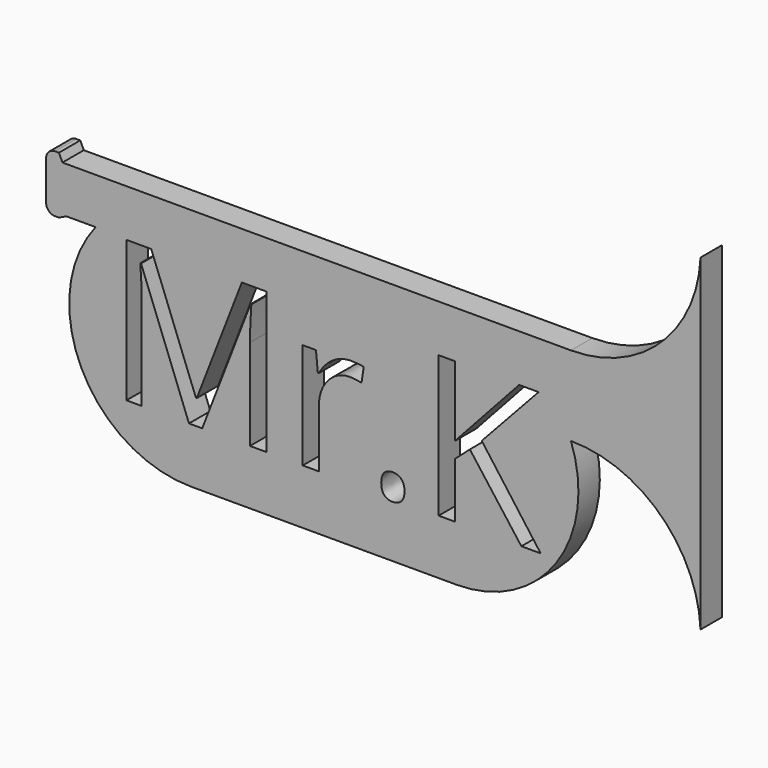
from build123d import *

# Parameters (mm, degrees)
F1_DEPTH     = 3
F2_TEXT_SIZE = 22.2222222222
F3_DEPTH     = 25


# Not quite as in the source:
# - Text() gives the source's letters only with a copy of the font that has no kerning and outlines rounded to 1/6400 em; it was checked with that copy


with BuildPart() as f1:
    # F0 (on Front) → F1 (new body)
    with BuildSketch(Plane.XZ):
        with BuildLine():
            Line((-13.9879264009, 8.4983842463), (-10.7078288449, 8.4983842463))
            ThreePointArc((-10.7078288449, 8.4983842463), (-12.3096819162, -5.9457433928), (0, -13.6704108706))
            Line((0, -13.6704108706), (29.832560569, -13.6704108706))
            ThreePointArc((29.832560569, -13.6704108706), (41.0439649972, -7.8220549805), (42.6626390029, 4.7190275219))
            ThreePointArc((42.6626390029, 4.7190275219), (52.7277631814, 0.6811115523), (57.2114773095, -9.193492122))
            Line((57.2114773095, -9.193492122), (57.2114773095, 27.5829305145))
            ThreePointArc((57.2114773095, 27.5829305145), (52.7277631814, 17.7083268402), (42.6626390029, 13.6704108706))
            Line((42.6626390029, 13.6704108706), (29.832560569, 13.6704108706))
            Line((29.832560569, 13.6704108706), (0, 13.6704108706))
            Line((0, 13.6704108706), (-14.4307379611, 13.6704108706))
            Line((-14.4307379611, 13.6704108706), (-14.8297163701, 14.5122008398))
            Line((-14.8297163701, 14.5122008398), (-15.268201828, 14.5122008398))
            ThreePointArc((-15.268201828, 14.5122008398), (-15.9753086092, 14.219307621), (-16.268201828, 13.5122008398))
            Line((-16.268201828, 13.5122008398), (-16.268201828, 9.0994058373))
            ThreePointArc((-16.268201828, 9.0994058373), (-15.9753086092, 8.3922990562), (-15.268201828, 8.0994058373))
            Line((-15.268201828, 8.0994058373), (-14.8297163701, 8.0994058373))
            Line((-14.8297163701, 8.0994058373), (-13.9879264009, 8.4983842463))
        make_face()
    extrude(amount=F1_DEPTH)

    # F2 (on face) → F3 (cut)
    with BuildSketch(Plane.XZ.offset(3)):
        with Locations((-9.423628505, -7.4973227103)):
            Text('Mr.K', F2_TEXT_SIZE, font='Open Sans', text_align=(TextAlign.LEFT, TextAlign.BOTTOM))
    extrude(amount=-F3_DEPTH, mode=Mode.SUBTRACT)


solid = f1.part
